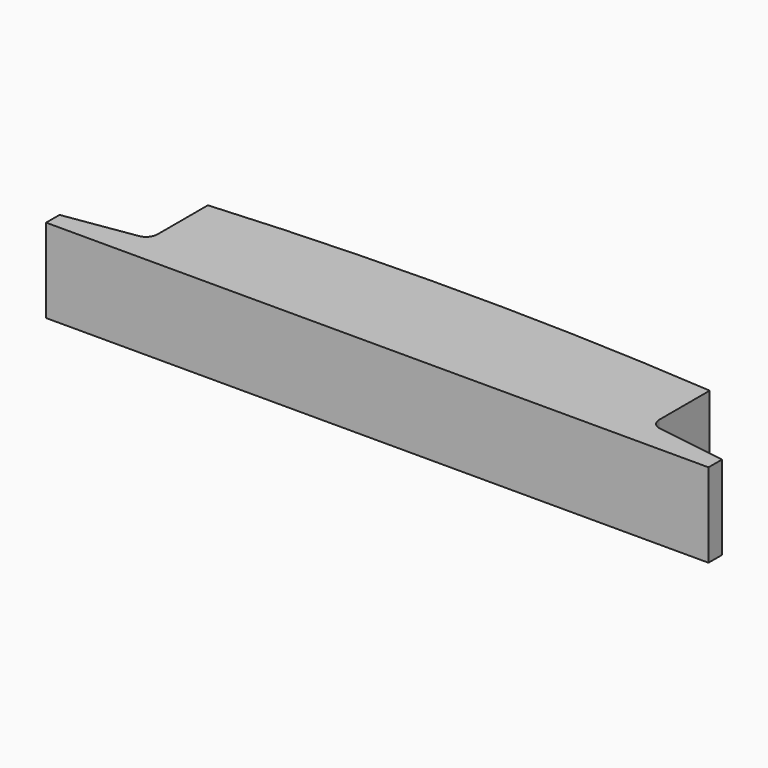
from build123d import *

# Parameters (mm, degrees)
F1_DEPTH = 3.75


# Not quite as in the source:
# - a feature of the source that left no trace in its solid (it failed there, or was rolled back) is left out


with BuildPart() as f1:
    # F0 (on Top) → F1 (new body)
    with BuildSketch(Plane.XY):
        with BuildLine():
            Line((11.2, 144.2591021933), (11.2, 147.0741649645))
            ThreePointArc((11.2, 147.0741649645), (0, 147.5), (-11.2, 147.0741649645))
            Line((-11.2, 147.0741649645), (-11.2, 144.2591021933))
            ThreePointArc((-11.2, 144.2591021933), (-11.3222315822, 143.9291191636), (-11.6299352058, 143.7583917795))
            Line((-11.6299352058, 143.7583917795), (-14.7849675268, 143.2757224802))
            Line((-14.7849675268, 143.2757224802), (-14.7849675268, 142.5268018024))
            Line((-14.7849675268, 142.5268018024), (-11.2, 142.5268018024))
            Line((-11.2, 142.5268018024), (11.2, 142.5268018024))
            Line((11.2, 142.5268018024), (14.7849675268, 142.5268018024))
            Line((14.7849675268, 142.5268018024), (14.7849675268, 143.2757224802))
            Line((14.7849675268, 143.2757224802), (11.6299352058, 143.7583917795))
            ThreePointArc((11.6299352058, 143.7583917795), (11.3222315822, 143.9291191636), (11.2, 144.2591021933))
        make_face()
    extrude(amount=F1_DEPTH)


solid = f1.part
